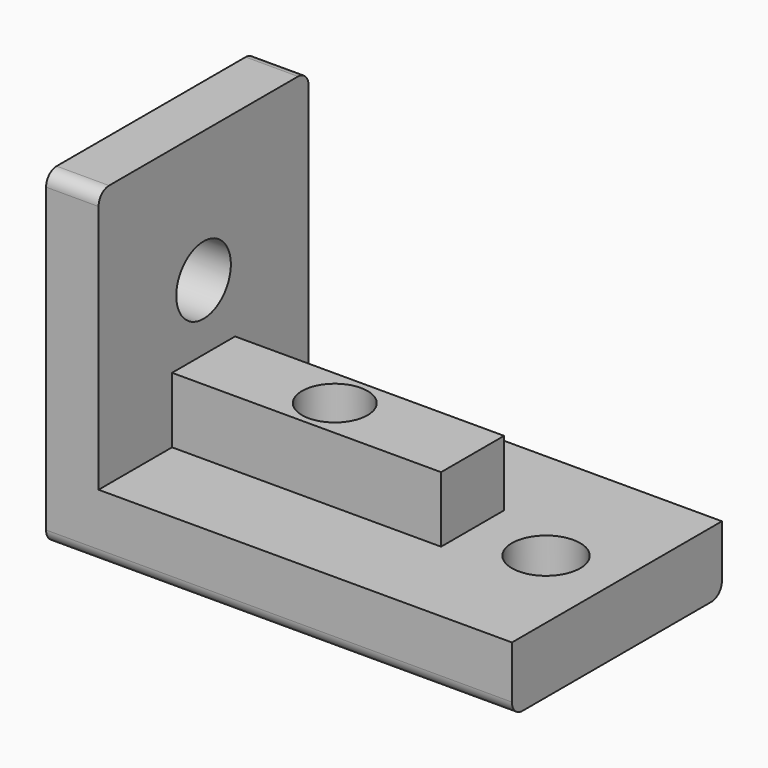
from build123d import *

# Parameters (mm, degrees)
F0_W      = 31.5
F0_H      = 20
F1_DEPTH  = 5
F2_W      = 31.5
F2_H      = 6
F3_DEPTH  = 5
F4_R      = 2.5
F5_DEPTH  = 25
F6_W      = 11.2
F6_H      = 6
F7_DEPTH  = 5
F8_R      = 2.6
F9_DEPTH  = 5
F10_R     = 2.6
F11_DEPTH = 4
F12_R     = 1


# Not quite as in the source:
# - a fillet or chamfer that OpenCascade refuses, or shapes differently, is made with other operations: its cross-section is extruded or revolved along the edge and cut away or added
# - a feature names something its author has since deleted; it is built from what else it names


with BuildPart() as f1:
    # F0 (on Top) → F1 (new body)
    with BuildSketch(Plane.XY):
        with Locations((15.75, 0)):
            Rectangle(F0_W, F0_H)
    extrude(amount=F1_DEPTH)

    # F2 (on face) → F3 (join)
    with BuildSketch(Plane.XY.offset(5)):
        with Locations((15.75, 0)):
            Rectangle(F2_W, F2_H)
    extrude(amount=F3_DEPTH)

    # F4 (on face) → F5 (cut)
    with BuildSketch(Plane.XY.offset(10)):
        with Locations((10, 0)):
            Circle(F4_R)
    extrude(amount=-F5_DEPTH, mode=Mode.SUBTRACT)

    # F6 (on face) → F7 (cut, through all)
    with BuildSketch(Plane.XY.offset(10)):
        with Locations((26.1, 0)):
            Rectangle(F6_W, F6_H)
    extrude(amount=-F7_DEPTH, mode=Mode.SUBTRACT)

    # F8 (on face) → F9 (cut, through all)
    with BuildSketch(Plane.XY.offset(5)):
        with Locations((26.1, 0)):
            Circle(F8_R)
    extrude(amount=-F9_DEPTH, mode=Mode.SUBTRACT)

    # F10 (on face) → F11 (join)
    with BuildSketch(Plane(origin=(0, 0, 0), x_dir=(0, -1, 0), z_dir=(-1, 0, 0))):
        Polygon((-10, 25), (-10, 5), (-3, 5), (-3, 10), (3, 10), (3, 5), (10, 5), (10, 25), align=None)
        with Locations((0, 15)):
            Circle(F10_R, mode=Mode.SUBTRACT)
        Polygon((-10, 5), (-10, 0), (10, 0), (10, 5), (3, 5), (3, 10), (-3, 10), (-3, 5), align=None)
    extrude(amount=F11_DEPTH)

    # F12
    f12_edges = [f1.edges().sort_by_distance(p)[0] for p in [
        (-2, -10, 25),
        (-2, 10, 25),
        (13.75, -10, 0),
        (13.75, 10, 0),
    ]]
    fillet(f12_edges, radius=F12_R)

    # F13: chamfer of 0.5 x 0.2886751346 on 1 edges, made by hand

    # F13_s1 → F13_t2 (revolve, cut)
    with BuildSketch(Plane.XZ):
        Polygon((12.7886751346, 0), (12.5, 0.5), (12.5, 0), align=None)
    revolve(axis=Axis((10, 0, 0), (0, 0, 1)), mode=Mode.SUBTRACT)


solid = f1.part
